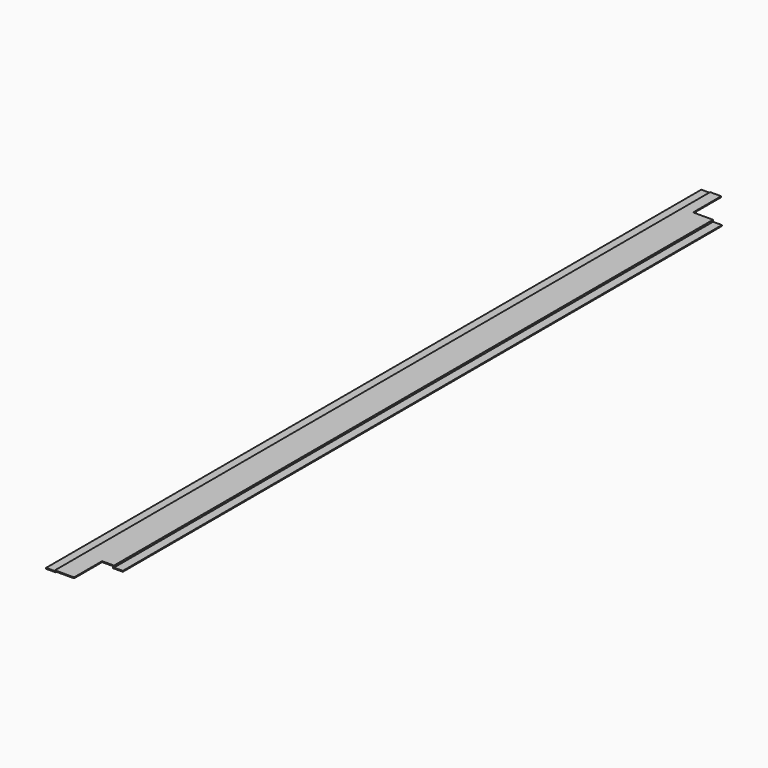
from build123d import *

# Parameters (mm, degrees)
F1_DEPTH = 2312
F2_W     = 56.23
F2_H     = 99
F2_W_2   = 25
F2_W_3   = 33.5
F3_DEPTH = 7.501


# Not quite as in the source:
# - a feature names something its author has since deleted; it is built from what else it names


with BuildPart() as f1:
    # F0 (on Front) → F1 (new body)
    with BuildSketch(Plane.XZ):
        Polygon((87.5, 0), (0, 0), (0, -2), (-25, -2), (-25, -4.5), (2.5, -4.5), (2.5, -2.5), (85, -2.5), (85, -7.5), (112.5, -7.5), (112.5, -5), (87.5, -5), align=None)
    extrude(amount=F1_DEPTH)

    # F2 (on face) → F3 (cut, through all)
    with BuildSketch(Plane.XY):
        with Locations((59.385, -49.5)):
            Rectangle(F2_W, F2_H)
        with Locations((100, -49.5)):
            Rectangle(F2_W_2, F2_H)
        Polygon((127.1371338549, -2213), (87.5, -2213), (87.5, -2312), (54, -2312), (54, -2342.1576023102), (127.1371338549, -2342.1576023102), align=None)
        with Locations((70.75, -2262.5)):
            Rectangle(F2_W_3, F2_H)
    extrude(amount=-F3_DEPTH, mode=Mode.SUBTRACT)


solid = f1.part
